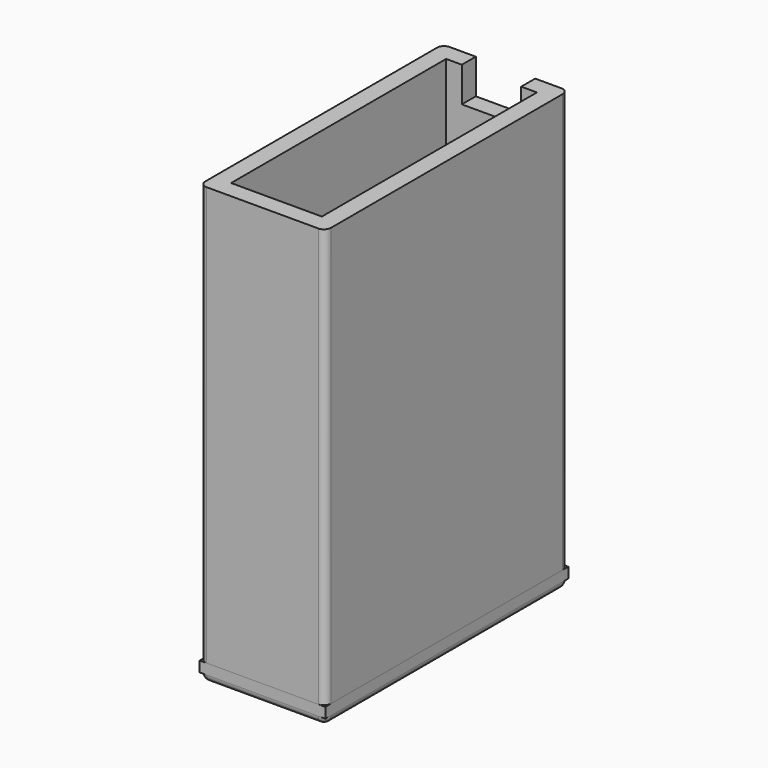
from build123d import *

# Parameters (mm, degrees)
F0_W     = 35.9999979138
F0_H     = 86.9999979138
F0_W_2   = 26
F0_H_2   = 77
F1_DEPTH = 120
F2_DEPTH = 5
F3_R     = 2
F5_W     = 17
F5_H     = 10
F6_DEPTH = 25
F7_DEPTH = 2
F0_W_3   = 21
F0_H_3   = 74
F8_DEPTH = 3


with BuildPart() as f1:
    # F0 (on Top) → F1 (new body)
    with BuildSketch(Plane.XY):
        Rectangle(F0_W, F0_H)
        Rectangle(F0_W_2, F0_H_2, mode=Mode.SUBTRACT)
    extrude(amount=F1_DEPTH)

    # F0 (on Top) → F2 (join)
    with BuildSketch(Plane.XY):
        Rectangle(F0_W, F0_H)
        Rectangle(F0_W_2, F0_H_2, mode=Mode.SUBTRACT)
        Rectangle(F0_W_2, F0_H_2)
        Polygon((12.5, 38), (12.5, -38), (-12.5, -38), (-12.5, 38), (-10.5, 38), (10.5, 38), align=None, mode=Mode.SUBTRACT)
    extrude(amount=-F2_DEPTH)

    # F3
    f3_edges = [f1.edges().sort_by_distance(p)[0] for p in [
        (0, 43.499999, -5),
        (0, -43.499999, -5),
        (-17.999999, -43.499999, 57.5),
        (17.999999, 0, -5),
        (17.999999, -43.499999, 57.5),
        (17.999999, 43.499999, 57.5),
        (-17.999999, 0, -5),
        (-17.999999, 43.499999, 57.5),
    ]]
    fillet(f3_edges, radius=F3_R)

    # F5 (on face) → F6 (cut)
    with BuildSketch(Plane(origin=(0, 43.4999989569, 0), x_dir=(-1, 0, 0), z_dir=(0, 1, 0))):
        with Locations((0, 115)):
            Rectangle(F5_W, F5_H)
    extrude(amount=-F6_DEPTH, mode=Mode.SUBTRACT)


with BuildPart() as f7:
    # F0 (on Top) → F7 (new body)
    with BuildSketch(Plane.XY):
        Polygon((-12.5, -38), (12.5, -38), (12.5, 38), (10.5, 38), (10.5, -36), (-10.5, -36), (-10.5, 38), (-12.5, 38), align=None)
    extrude(amount=F7_DEPTH)

    # F0 (on Top) → F8 (join)
    with BuildSketch(Plane.XY):
        Rectangle(F0_W, F0_H)
        Rectangle(F0_W_2, F0_H_2, mode=Mode.SUBTRACT)
        Rectangle(F0_W_2, F0_H_2)
        Polygon((12.5, 38), (12.5, -38), (-12.5, -38), (-12.5, 38), (-10.5, 38), (10.5, 38), align=None, mode=Mode.SUBTRACT)
        with Locations((0, 1)):
            Rectangle(F0_W_3, F0_H_3)
        Polygon((-12.5, -38), (12.5, -38), (12.5, 38), (10.5, 38), (10.5, -36), (-10.5, -36), (-10.5, 38), (-12.5, 38), align=None)
    extrude(amount=-F8_DEPTH)


solid = Compound([f1.part, f7.part])
